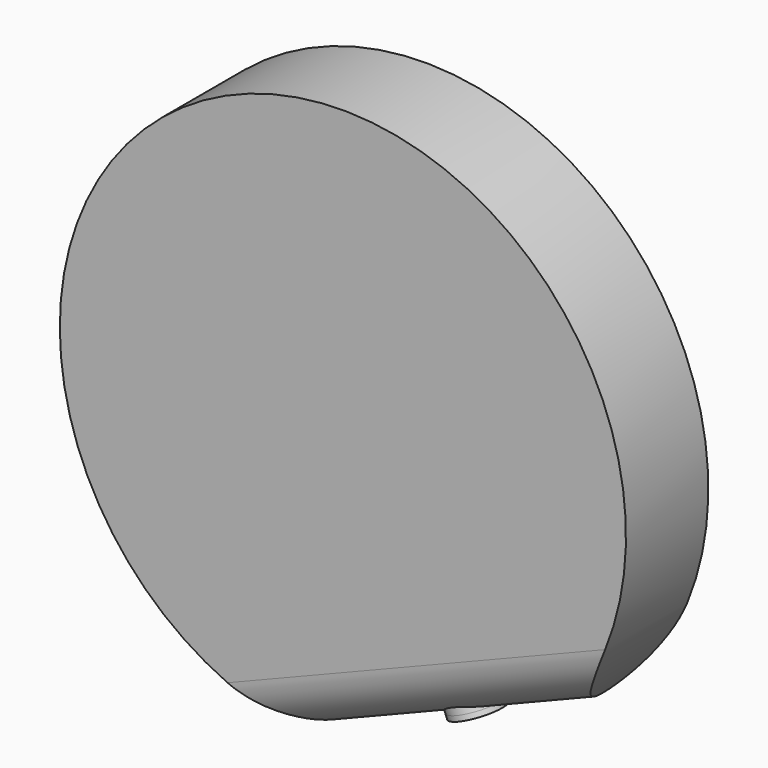
from build123d import *

# Parameters (mm, degrees)
F1_DEPTH     = 10
F2_R         = 2.5
F3_DEPTH     = 0.5
F4_T4_DEPTH  = 51.44253063
F4_S5_R      = 2.5
F4_T6_DEPTH  = 29
F4_T10_DEPTH = 51.44253063
F4_S11_R     = 2.5
F4_T12_DEPTH = 29


# Not quite as in the source:
# - a fillet or chamfer that OpenCascade refuses, or shapes differently, is made with other operations: its cross-section is extruded or revolved along the edge and cut away or added


with BuildPart() as f1:
    # F0 (on Front) → F1 (new body)
    with BuildSketch(Plane.XZ):
        with BuildLine():
            Line((-18.7246046442, 1.2957563709), (5.805945114, 11.1679169591))
            ThreePointArc((5.805945114, 11.1679169591), (-25.7288225372, 54.1130726963), (-18.7246046442, 1.2957563709))
        make_face()
    extrude(amount=F1_DEPTH)

    # F2 (on face) → F3 (join)
    with BuildSketch(Plane(origin=(-3.0587265768, 0, 7.6003873539), x_dir=(0.9276929694, 0, 0.3733440164), z_dir=(0.3733440164, 0, -0.9276929694))):
        with Locations((-3.6656558802, 4.9999994226)):
            Circle(F2_R)
    extrude(amount=F3_DEPTH)

    # F4: fillet of radius 5 on 2 edges, made by hand


with BuildPart() as f4_tool2:
    # F4_s3 → F4_t4 (new body)
    with BuildSketch(Plane(origin=(-27.2620401847, 0, -10.9714311875), x_dir=(0, 1, 0), z_dir=(0.9276929694, 0, 0.3733440164))):
        with BuildLine():
            ThreePointArc((-5, 8.192783178), (-8.5355339059, 9.657249272), (-10, 13.192783178))
            Line((-10, 13.192783178), (-10, 8.192783178))
            Line((-10, 8.192783178), (-5, 8.192783178))
        make_face()
    extrude(amount=F4_T4_DEPTH)

    # F4_s5 → F4_t6 (cut, symmetric)
    with BuildSketch(Plane(origin=(-3.9947809751, 0, 9.9263147724), x_dir=(0, 1, 0), z_dir=(-0.3733440164, 0, 0.9276929694))):
        with Locations((-4.9999994226, 3.6656558802)):
            Circle(F4_S5_R)
    extrude(amount=F4_T6_DEPTH, both=True, mode=Mode.SUBTRACT)


with BuildPart() as f1_1:
    add(f1.part)

    # F4_t1: cut F4_tool2
    add(f4_tool2.part, mode=Mode.SUBTRACT)


with BuildPart() as f4_tool8:
    # F4_s9 → F4_t10 (new body)
    with BuildSketch(Plane(origin=(-27.2620401847, 0, -10.9714311875), x_dir=(0, 1, 0), z_dir=(0.9276929694, 0, 0.3733440164))):
        with BuildLine():
            ThreePointArc((-5, 8.192783178), (-1.4644660941, 9.657249272), (0, 13.192783178))
            Line((0, 13.192783178), (0, 8.192783178))
            Line((0, 8.192783178), (-5, 8.192783178))
        make_face()
    extrude(amount=F4_T10_DEPTH)

    # F4_s11 → F4_t12 (cut, symmetric)
    with BuildSketch(Plane(origin=(-3.9947809751, 0, 9.9263147724), x_dir=(0, 1, 0), z_dir=(-0.3733440164, 0, 0.9276929694))):
        with Locations((-4.9999994226, 3.6656558802)):
            Circle(F4_S11_R)
    extrude(amount=F4_T12_DEPTH, both=True, mode=Mode.SUBTRACT)


with BuildPart() as f1_2:
    add(f1_1.part)

    # F4_t7: cut F4_tool8
    add(f4_tool8.part, mode=Mode.SUBTRACT)


solid = f1_2.part
